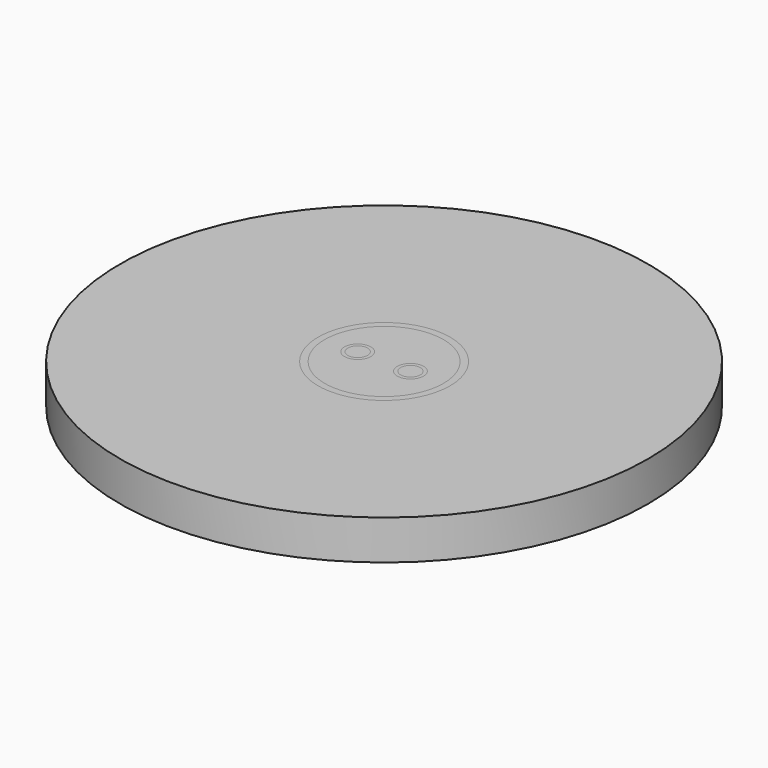
from build123d import *

# Parameters (mm, degrees)
F0_R      = 20
F0_R_2    = 5.5
F1_DEPTH  = 3
F2_R      = 5.5
F2_R_2    = 5
F3_DEPTH  = 6
F4_R      = 5
F4_R_2    = 4.5
F5_DEPTH  = 6
F6_R      = 4.5
F7_DEPTH  = 6
F8_R      = 1
F9_DEPTH  = 1
F11_R     = 1
F11_R_2   = 0.75
F12_DEPTH = 1
F13_R     = 0.75
F14_DEPTH = 9
F16_DEPTH = 3
F17_W     = 6.3846809013
F17_H     = 1
F18_DEPTH = 12.5
F19_W     = 1.7936326425
F19_H     = 0.7
F20_DEPTH = 12.5
F10_R     = 1
F21_DEPTH = 1
F22_R     = 1
F22_R_2   = 0.75
F23_DEPTH = 1
F24_R     = 0.75
F25_DEPTH = 25


with BuildPart() as f1:
    # F0 (on Top) → F1 (new body)
    with BuildSketch(Plane.XY):
        Circle(F0_R)
        Circle(F0_R_2, mode=Mode.SUBTRACT)
    extrude(amount=F1_DEPTH)

    # F2 (on face) → F3 (join)
    with BuildSketch(Plane.XY.offset(3)):
        Circle(F2_R)
        Circle(F2_R_2, mode=Mode.SUBTRACT)
    extrude(amount=-F3_DEPTH)

    # F17 (on Right) → F18 (cut, symmetric)
    with BuildSketch(Plane.YZ):
        with Locations((-2.9923404506, -9.5)):
            Rectangle(F17_W, F17_H)
    extrude(amount=F18_DEPTH, both=True, mode=Mode.SUBTRACT)


with BuildPart() as f5:
    # F4 (on face) → F5 (new body)
    with BuildSketch(Plane.XY.offset(3)):
        Circle(F4_R)
        Circle(F4_R_2, mode=Mode.SUBTRACT)
    extrude(amount=-F5_DEPTH)


with BuildPart() as f7:
    # F6 (on face) → F7 (new body)
    with BuildSketch(Plane.XY.offset(3)):
        Circle(F6_R)
    extrude(amount=-F7_DEPTH)

    # F8 (on face) → F9 (cut)
    with BuildSketch(Plane.XY.offset(3)):
        with Locations((-2, 0)):
            Circle(F8_R)
        with Locations((2, 0)):
            Circle(F8_R)
    extrude(amount=-F9_DEPTH, mode=Mode.SUBTRACT)

    # F10 (on face) → F21 (cut)
    with BuildSketch(Plane(origin=(0, 0, -3), x_dir=(1, 0, 0), z_dir=(0, 0, -1))):
        with Locations((-2, 0)):
            Circle(F10_R)
        with Locations((2, 0)):
            Circle(F10_R)
    extrude(amount=-F21_DEPTH, mode=Mode.SUBTRACT)

    # F24 (on face) → F25 (cut)
    with BuildSketch(Plane.XY.offset(2)):
        with Locations((-2, 0)):
            Circle(F24_R)
        with Locations((2, 0)):
            Circle(F24_R)
    extrude(amount=-F25_DEPTH, mode=Mode.SUBTRACT)


with BuildPart() as f12:
    # F11 (on face) → F12 (new body)
    with BuildSketch(Plane.XY.offset(3)):
        with Locations((-2, 0)):
            Circle(F11_R)
        with Locations((-2, 0)):
            Circle(F11_R_2, mode=Mode.SUBTRACT)
    extrude(amount=-F12_DEPTH)


with BuildPart() as f12b:
    # F11 (on face) → F12, piece 2 (new body)
    with BuildSketch(Plane.XY.offset(3)):
        with Locations((2, 0)):
            Circle(F11_R)
        with Locations((2, 0)):
            Circle(F11_R_2, mode=Mode.SUBTRACT)
    extrude(amount=-F12_DEPTH)


with BuildPart() as f14:
    # F13 (on face) → F14 (new body)
    with BuildSketch(Plane.XY.offset(3)):
        with Locations((-2, 0)):
            Circle(F13_R)
    extrude(amount=-F14_DEPTH)


with BuildPart() as f14b:
    # F13 (on face) → F14, piece 2 (new body)
    with BuildSketch(Plane.XY.offset(3)):
        with Locations((2, 0)):
            Circle(F13_R)
    extrude(amount=-F14_DEPTH)


with BuildPart() as f16_tool:
    # F15 (on face) → F16 (new body)
    with BuildSketch(Plane(origin=(0, 0, -6), x_dir=(1, 0, 0), z_dir=(0, 0, -1))):
        with BuildLine():
            Line((-1.4343145751, 0.2), (-1.2771583853, 0.2))
            ThreePointArc((-1.2771583853, 0.2), (-2, 0.75), (-2.7228416147, 0.2))
            Line((-2.7228416147, 0.2), (-2.5656854249, 0.2))
            ThreePointArc((-2.5656854249, 0.2), (-2, -0.6), (-1.4343145751, 0.2))
        make_face()
        with BuildLine():
            Line((2.5656854249, 0.2), (2.7228416147, 0.2))
            ThreePointArc((2.7228416147, 0.2), (2, 0.75), (1.2771583853, 0.2))
            Line((1.2771583853, 0.2), (1.4343145751, 0.2))
            ThreePointArc((1.4343145751, 0.2), (2, -0.6), (2.5656854249, 0.2))
        make_face()
    extrude(amount=-F16_DEPTH)


with BuildPart() as f14_1:
    add(f14.part)

    # F16: cut by f16_tool
    add(f16_tool.part, mode=Mode.SUBTRACT)


with BuildPart() as f14b_1:
    add(f14b.part)

    # F16: cut by f16_tool
    add(f16_tool.part, mode=Mode.SUBTRACT)


with BuildPart() as f20_tool:
    # F19 (on Right) → F20 (new body, symmetric)
    with BuildSketch(Plane.YZ):
        with Locations((-0.5968163213, -3.35)):
            Rectangle(F19_W, F19_H)
    extrude(amount=F20_DEPTH, both=True)


with BuildPart() as f14_2:
    add(f14_1.part)

    # F20: cut by f20_tool
    add(f20_tool.part, mode=Mode.SUBTRACT)


with BuildPart() as f14b_2:
    add(f14b_1.part)

    # F20: cut by f20_tool
    add(f20_tool.part, mode=Mode.SUBTRACT)


with BuildPart() as f23:
    # F22 (on face) → F23 (new body)
    with BuildSketch(Plane(origin=(0, 0, -3), x_dir=(1, 0, 0), z_dir=(0, 0, -1))):
        with Locations((-2, 0)):
            Circle(F22_R)
        with Locations((-2, 0)):
            Circle(F22_R_2, mode=Mode.SUBTRACT)
    extrude(amount=-F23_DEPTH)


with BuildPart() as f23b:
    # F22 (on face) → F23, piece 2 (new body)
    with BuildSketch(Plane(origin=(0, 0, -3), x_dir=(1, 0, 0), z_dir=(0, 0, -1))):
        with Locations((2, 0)):
            Circle(F22_R)
        with Locations((2, 0)):
            Circle(F22_R_2, mode=Mode.SUBTRACT)
    extrude(amount=-F23_DEPTH)


solid = Compound([f1.part, f5.part, f7.part, f12.part, f12b.part, f14_2.part, f14b_2.part, f23.part, f23b.part])
